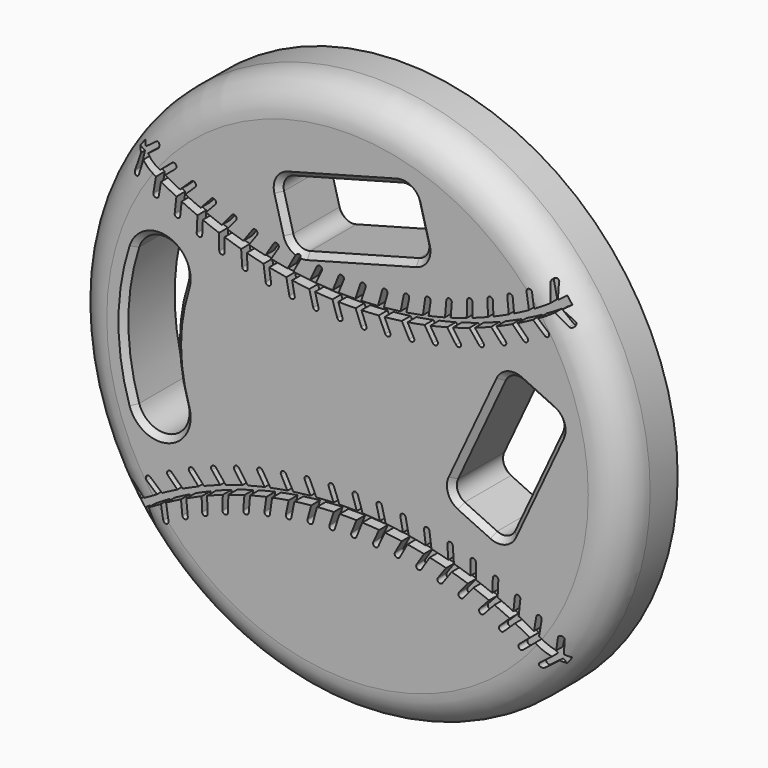
from build123d import *

# Parameters (mm, degrees)
F0_R          = 12.7
F1_DEPTH      = 3.175
F2_SIZE       = 0.254
F5_DEPTH      = 0.508
F7_DEPTH      = 0.508
F9_DEPTH      = 0.508
F14_DEPTH     = 25.4
F15_SIZE      = 0.254
F17_DEPTH     = 25.4
F18_T1_DEPTH  = 1.651
F18_T3_DEPTH  = 5.207
F18_T5_DEPTH  = 1.651
F18_T7_DEPTH  = 5.207
F18_T10_ANGLE = 90
F18_T12_ANGLE = 90
F18_T14_ANGLE = 90
F18_T16_ANGLE = 90
F18_T18_ANGLE = 90
F18_T20_ANGLE = 90
F18_T22_ANGLE = 90
F18_T24_ANGLE = 90


# Not quite as in the source:
# - a fillet or chamfer that OpenCascade refuses, or shapes differently, is made with other operations: its cross-section is extruded or revolved along the edge and cut away or added
# - ends of sketch curves that miss each other by under 0.0002 mm in the source are joined


with BuildPart() as f1:
    # F0 (on Front) → F1 (new body)
    with BuildSketch(Plane.XZ):
        Circle(F0_R)
        with BuildLine():
            ThreePointArc((-9.818145271, -3.175), (-10.31875, 0), (-9.818145271, 3.175))
            ThreePointArc((-9.818145271, 3.175), (-8.3189362013, 3.941516762), (-7.5524194392, 2.4423076923))
            ThreePointArc((-7.5524194392, 2.4423076923), (-7.9375, 0), (-7.5524194392, -2.4423076923))
            ThreePointArc((-7.5524194392, -2.4423076923), (-8.3189362013, -3.941516762), (-9.818145271, -3.175))
        make_face(mode=Mode.SUBTRACT)
    extrude(amount=F1_DEPTH)

    # F2
    f2_edges = [f1.edges().sort_by_distance(p)[0] for p in [
        (-8.318936, -3.175, -3.941517),
        (-7.9375, -3.175, 0),
        (-7.9375, 0, 0),
    ]]
    chamfer(f2_edges, length=F2_SIZE)

    # F4 (on face) → F5 (cut)
    with BuildSketch(Plane.XZ.offset(3.175)):
        with BuildLine():
            ThreePointArc((10.0903170963, 7.7120361057), (0, 4.4873333333), (-10.0903170963, 7.7120361057))
            ThreePointArc((-10.0903170963, 7.7120361057), (-10.204882315, 7.5597868314), (-10.3171505, 7.4058359123))
            ThreePointArc((-10.3171505, 7.4058359123), (0, 4.1063333333), (10.3171505, 7.4058359123))
            ThreePointArc((10.3171505, 7.4058359123), (10.204882315, 7.5597868314), (10.0903170963, 7.7120361057))
        make_face()
        with BuildLine():
            ThreePointArc((-10.3171505, -7.4058359123), (-10.204882315, -7.5597868314), (-10.0903170963, -7.7120361057))
            ThreePointArc((-10.0903170963, -7.7120361057), (0, -4.4873333333), (10.0903170963, -7.7120361057))
            ThreePointArc((10.0903170963, -7.7120361057), (10.204882315, -7.5597868314), (10.3171505, -7.4058359123))
            ThreePointArc((10.3171505, -7.4058359123), (0, -4.1063333333), (-10.3171505, -7.4058359123))
        make_face()
    extrude(amount=-F5_DEPTH, mode=Mode.SUBTRACT)

    # F6 (on face) → F7 (cut)
    with BuildSketch(Plane.XZ.offset(3.175)):
        with BuildLine():
            Line((8.9655202832, -7.7774051542), (9.7084275034, -7.2188150469))
            ThreePointArc((9.7084275034, -7.2188150469), (9.5954418436, -7.1446517893), (9.481889674, -7.0713588641))
            Line((9.481889674, -7.0713588641), (8.8128738495, -7.5743902131))
            ThreePointArc((8.8128738495, -7.5743902131), (8.7876895958, -7.7522209005), (8.9655202832, -7.7774051542))
        make_face()
        with BuildLine():
            Line((-9.1205047211, -7.8770944945), (-9.3207214809, -6.9694341534))
            ThreePointArc((-9.3207214809, -6.9694341534), (-9.4350615627, -7.0414917261), (-9.5488446034, -7.1144257218))
            Line((-9.5488446034, -7.1144257218), (-9.3685418994, -7.931807913))
            ThreePointArc((-9.3685418994, -7.931807913), (-9.217166601, -8.0284697929), (-9.1205047211, -7.8770944945))
        make_face()
        with BuildLine():
            ThreePointArc((-9.5488446034, -7.1144257218), (-9.4350615627, -7.0414917261), (-9.3207214809, -6.9694341534))
            Line((-9.3207214809, -6.9694341534), (-10.0499520862, -6.4086497383))
            ThreePointArc((-10.0499520862, -6.4086497383), (-10.2280453511, -6.4319046086), (-10.2047904808, -6.6099978735))
            Line((-10.2047904808, -6.6099978735), (-9.5488446034, -7.1144257218))
        make_face()
        with BuildLine():
            Line((-8.2616111371, -7.3540137205), (-8.4068864974, -6.4359564699))
            ThreePointArc((-8.4068864974, -6.4359564699), (-8.5253526153, -6.5010081955), (-8.6433154009, -6.5669682539))
            Line((-8.6433154009, -6.5669682539), (-8.5124894884, -7.3937132522))
            ThreePointArc((-8.5124894884, -7.3937132522), (-8.3672005469, -7.4993026621), (-8.2616111371, -7.3540137205))
        make_face()
        with BuildLine():
            ThreePointArc((-8.6433154009, -6.5669682539), (-8.5253526153, -6.5010081955), (-8.4068864974, -6.4359564699))
            Line((-8.4068864974, -6.4359564699), (-9.1010766453, -5.8323369918))
            ThreePointArc((-9.1010766453, -5.8323369918), (-9.280245996, -5.8448407425), (-9.2677422452, -6.0240100932))
            Line((-9.2677422452, -6.0240100932), (-8.6433154009, -6.5669682539))
        make_face()
        with BuildLine():
            Line((-7.3728180575, -6.8835261579), (-7.4626262541, -5.9583945275))
            ThreePointArc((-7.4626262541, -5.9583945275), (-7.5847896689, -6.0162049781), (-7.7065052817, -6.0749523839))
            Line((-7.7065052817, -6.0749523839), (-7.6256296312, -6.9080681266))
            ThreePointArc((-7.6256296312, -6.9080681266), (-7.48695286, -7.0222029291), (-7.3728180575, -6.8835261579))
        make_face()
        with BuildLine():
            ThreePointArc((-7.7065052817, -6.0749523839), (-7.5847896689, -6.0162049781), (-7.4626262541, -5.9583945275))
            Line((-7.4626262541, -5.9583945275), (-8.1192636096, -5.3141245382))
            ThreePointArc((-8.1192636096, -5.3141245382), (-8.2988606164, -5.3158319172), (-8.2971532374, -5.495428924))
            Line((-8.2971532374, -5.495428924), (-7.7065052817, -6.0749523839))
        make_face()
        with BuildLine():
            Line((-6.4573421027, -6.4673345424), (-6.4913581118, -5.5384766648))
            ThreePointArc((-6.4913581118, -5.5384766648), (-6.6167767033, -5.5888366191), (-6.7418046438, -5.6401587604))
            Line((-6.7418046438, -5.6401587604), (-6.7111719514, -6.4766301285))
            ThreePointArc((-6.7111719514, -6.4766301285), (-6.5796092339, -6.5988972598), (-6.4573421027, -6.4673345424))
        make_face()
        with BuildLine():
            ThreePointArc((-6.7418046438, -5.6401587604), (-6.6167767033, -5.5888366191), (-6.4913581118, -5.5384766648))
            Line((-6.4913581118, -5.5384766648), (-7.1080662467, -4.8558878338))
            ThreePointArc((-7.1080662467, -4.8558878338), (-7.2874409323, -4.8467926619), (-7.2965361041, -5.0261673476))
            Line((-7.2965361041, -5.0261673476), (-6.7418046438, -5.6401587604))
        make_face()
        with BuildLine():
            Line((-5.5184964603, -6.1069451079), (-5.4965971749, -5.1777226012))
            ThreePointArc((-5.4965971749, -5.1777226012), (-5.6248170423, -5.2204498023), (-5.7527048234, -5.2641609397))
            Line((-5.7527048234, -5.2641609397), (-5.7724259515, -6.10096067))
            ThreePointArc((-5.7724259515, -6.10096067), (-5.6484534248, -6.2309176346), (-5.5184964603, -6.1069451079))
        make_face()
        with BuildLine():
            ThreePointArc((-5.7527048234, -5.2641609397), (-5.6248170423, -5.2204498023), (-5.4965971749, -5.1777226012))
            Line((-5.4965971749, -5.1777226012), (-6.0711441684, -4.4592852774))
            ThreePointArc((-6.0711441684, -4.4592852774), (-6.2496473602, -4.439420471), (-6.2695121666, -4.6179236627))
            Line((-6.2695121666, -4.6179236627), (-5.7527048234, -5.2641609397))
        make_face()
        with BuildLine():
            Line((-4.559678895, -5.8036621355), (-4.4819435707, -4.8774379374))
            ThreePointArc((-4.4819435707, -4.8774379374), (-4.612500675, -4.9123777518), (-4.7427854596, -4.9483196908))
            Line((-4.7427854596, -4.9483196908), (-4.8127890357, -5.7824193317))
            ThreePointArc((-4.8127890357, -5.7824193317), (-4.6968553672, -5.9195958039), (-4.559678895, -5.8036621355))
        make_face()
        with BuildLine():
            ThreePointArc((-4.7427854596, -4.9483196908), (-4.612500675, -4.9123777518), (-4.4819435707, -4.8774379374))
            Line((-4.4819435707, -4.8774379374), (-5.0122500868, -4.1257522086))
            ThreePointArc((-5.0122500868, -4.1257522086), (-5.1892357659, -4.09518966), (-5.2197983146, -4.2721753391))
            Line((-5.2197983146, -4.2721753391), (-4.7427854596, -4.9483196908))
        make_face()
        with BuildLine():
            Line((-3.5843594519, -5.5585832327), (-3.4510694196, -4.63870943))
            ThreePointArc((-3.4510694196, -4.63870943), (-3.5834912631, -4.6657354074), (-3.7157015392, -4.6937780711))
            Line((-3.7157015392, -4.6937780711), (-3.8357342141, -5.5221589427))
            ThreePointArc((-3.8357342141, -5.5221589427), (-3.728258978, -5.6660584689), (-3.5843594519, -5.5585832327))
        make_face()
        with BuildLine():
            ThreePointArc((-3.7157015392, -4.6937780711), (-3.5834912631, -4.6657354074), (-3.4510694196, -4.63870943))
            Line((-3.4510694196, -4.63870943), (-3.9352162324, -3.8564957127))
            ThreePointArc((-3.9352162324, -3.8564957127), (-4.1100438722, -3.8153460305), (-4.1511935545, -3.9901736703))
            Line((-4.1511935545, -3.9901736703), (-3.7157015392, -4.6937780711))
        make_face()
        with BuildLine():
            Line((-2.5960678974, -5.3725953618), (-2.4077055454, -4.4624010583))
            ThreePointArc((-2.4077055454, -4.4624010583), (-2.541512882, -4.4814153893), (-2.6751701689, -4.5014572888))
            Line((-2.6751701689, -4.5014572888), (-2.8447975339, -5.3211214082))
            ThreePointArc((-2.8447975339, -5.3211214082), (-2.7461696925, -5.4712232033), (-2.5960678974, -5.3725953618))
        make_face()
        with BuildLine():
            ThreePointArc((-2.6751701689, -4.5014572888), (-2.541512882, -4.4814153893), (-2.4077055454, -4.4624010583))
            Line((-2.4077055454, -4.4624010583), (-2.8439404852, -3.6524902526))
            ThreePointArc((-2.8439404852, -3.6524902526), (-3.0159773692, -3.6009023611), (-3.0675652608, -3.772939245))
            Line((-3.0675652608, -3.772939245), (-2.6751701689, -4.5014572888))
        make_face()
        with BuildLine():
            Line((-1.5983809455, -5.246371629), (-1.3556279737, -4.3491508979))
            ThreePointArc((-1.3556279737, -4.3491508979), (-1.4903365427, -4.360084768), (-1.6249571231, -4.3720533698))
            Line((-1.6249571231, -4.3720533698), (-1.8435652819, -5.1800343006))
            ThreePointArc((-1.8435652819, -5.1800343006), (-1.7541417779, -5.335795133), (-1.5983809455, -5.246371629))
        make_face()
        with BuildLine():
            ThreePointArc((-1.6249571231, -4.3720533698), (-1.4903365427, -4.360084768), (-1.3556279737, -4.3491508979))
            Line((-1.3556279737, -4.3491508979), (-1.742372268, -3.514474142))
            ThreePointArc((-1.742372268, -3.514474142), (-1.9109957795, -3.4526347423), (-1.9728351792, -3.6212582538))
            Line((-1.9728351792, -3.6212582538), (-1.6249571231, -4.3720533698))
        make_face()
        with BuildLine():
            Line((-0.5949093127, -5.1803688492), (-0.2986442654, -4.2993688109))
            ThreePointArc((-0.2986442654, -4.2993688109), (-0.4337665448, -4.3021826495), (-0.5688632149, -4.3060346383))
            Line((-0.5688632149, -4.3060346383), (-0.8356610054, -5.0994082266))
            ThreePointArc((-0.8356610054, -5.0994082266), (-0.7557654704, -5.2602643843), (-0.5949093127, -5.1803688492))
        make_face()
        with BuildLine():
            ThreePointArc((-0.5688632149, -4.3060346383), (-0.4337665448, -4.3021826495), (-0.2986442654, -4.2993688109))
            Line((-0.2986442654, -4.2993688109), (-0.6344982526, -3.4429468734))
            ThreePointArc((-0.6344982526, -3.4429468734), (-0.7990981284, -3.3710797676), (-0.8709652341, -3.5356796434))
            Line((-0.8709652341, -3.5356796434), (-0.5688632149, -4.3060346383))
        make_face()
        with BuildLine():
            Line((0.4107153491, -5.1748258922), (0.7594202627, -4.3132349632))
            ThreePointArc((0.7594202627, -4.3132349632), (0.6243732923, -4.3079185867), (0.4892894591, -4.3036400218))
            Line((0.4892894591, -4.3036400218), (0.1752676015, -5.0795349789))
            ThreePointArc((0.1752676015, -5.0795349789), (0.2453460187, -5.2449043094), (0.4107153491, -5.1748258922))
        make_face()
        with BuildLine():
            ThreePointArc((0.4892894591, -4.3036400218), (0.6243732923, -4.3079185867), (0.7594202627, -4.3132349632))
            Line((0.7594202627, -4.3132349632), (0.4756720676, -3.43816731))
            ThreePointArc((0.4756720676, -3.43816731), (0.3156915289, -3.3565325916), (0.2340568106, -3.5165131303))
            Line((0.2340568106, -3.5165131303), (0.4892894591, -4.3036400218))
        make_face()
        with BuildLine():
            Line((1.414853596, -5.2297628184), (1.8147363823, -4.3906991719))
            ThreePointArc((1.8147363823, -4.3906991719), (1.6802534676, -4.3772718207), (1.5456713517, -4.3648781866))
            Line((1.5456713517, -4.3648781866), (1.1855618997, -5.1204864807))
            ThreePointArc((1.1855618997, -5.1204864807), (1.245569579, -5.2897704977), (1.414853596, -5.2297628184))
        make_face()
        with BuildLine():
            ThreePointArc((1.5456713517, -4.3648781866), (1.6802534676, -4.3772718207), (1.8147363823, -4.3906991719))
            Line((1.8147363823, -4.3906991719), (1.5841208889, -3.5001527497))
            ThreePointArc((1.5841208889, -3.5001527497), (1.4293386709, -3.4090458619), (1.3382317831, -3.5638280798))
            Line((1.3382317831, -3.5638280798), (1.5456713517, -4.3648781866))
        make_face()
        with BuildLine():
            Line((2.4138713637, -5.3449808064), (2.8634848117, -4.5314810872))
            ThreePointArc((2.8634848117, -4.5314810872), (2.7300526583, -4.5099913561), (2.5964593241, -4.4895275065))
            Line((2.5964593241, -4.4895275065), (2.1915655453, -5.2221145249))
            ThreePointArc((2.1915655453, -5.2221145249), (2.2412853137, -5.3947005748), (2.4138713637, -5.3449808064))
        make_face()
        with BuildLine():
            ThreePointArc((2.5964593241, -4.4895275065), (2.7300526583, -4.5099913561), (2.8634848117, -4.5314810872))
            Line((2.8634848117, -4.5314810872), (2.6868366377, -3.6286788616))
            ThreePointArc((2.6868366377, -3.6286788616), (2.5378129109, -3.5284295282), (2.4375635775, -3.677453255))
            Line((2.4375635775, -3.677453255), (2.5964593241, -4.4895275065))
        make_face()
        with BuildLine():
            Line((3.4041531191, -5.520062872), (3.9018700383, -4.7350712071))
            ThreePointArc((3.9018700383, -4.7350712071), (3.7699715489, -4.7055968693), (3.6378504824, -4.6771368646))
            Line((3.6378504824, -4.6771368646), (3.189637723, -5.3840513105))
            ThreePointArc((3.189637723, -5.3840513105), (3.2288896403, -5.5593147893), (3.4041531191, -5.520062872))
        make_face()
        with BuildLine():
            ThreePointArc((3.6378504824, -4.6771368646), (3.7699715489, -4.7055968693), (3.9018700383, -4.7350712071))
            Line((3.9018700383, -4.7350712071), (3.779828489, -3.8232804985))
            ThreePointArc((3.779828489, -3.8232804985), (3.6371025833, -3.7142515307), (3.5280736154, -3.8569774364))
            Line((3.5280736154, -3.8569774364), (3.6378504824, -4.6771368646))
        make_face()
        with BuildLine():
            Line((4.3821149457, -5.7543753779), (4.926134055, -5.0007327209))
            ThreePointArc((4.926134055, -5.0007327209), (4.7962465817, -4.9633804468), (4.6660759406, -4.9270272862))
            Line((4.6660759406, -4.9270272862), (4.1761663219, -5.6057107743))
            ThreePointArc((4.1761663219, -5.6057107743), (4.204808332, -5.783017388), (4.3821149457, -5.7543753779))
        make_face()
        with BuildLine():
            ThreePointArc((4.6660759406, -4.9270272862), (4.7962465817, -4.9633804468), (4.926134055, -5.0007327209))
            Line((4.926134055, -5.0007327209), (4.8591408094, -4.0832533801))
            ThreePointArc((4.8591408094, -4.0832533801), (4.7232292623, -3.9658393631), (4.6058152454, -4.1017509102))
            Line((4.6058152454, -4.1017509102), (4.6660759406, -4.9270272862))
        make_face()
        with BuildLine():
            Line((5.3442175139, -6.0470703267), (5.9325699604, -5.3275041765))
            ThreePointArc((5.9325699604, -5.3275041765), (5.8051635774, -5.2824091471), (5.6774144607, -5.2382943959))
            Line((5.6774144607, -5.2382943959), (5.1475810086, -5.8862907112))
            ThreePointArc((5.1475810086, -5.8862907112), (5.1655094535, -6.0649987716), (5.3442175139, -6.0470703267))
        make_face()
        with BuildLine():
            ThreePointArc((5.6774144607, -5.2382943959), (5.8051635774, -5.2824091471), (5.9325699604, -5.3275041765))
            Line((5.9325699604, -5.3275041765), (5.9208674729, -4.4076566415))
            ThreePointArc((5.9208674729, -4.4076566415), (5.7922621603, -4.2822825071), (5.6668880259, -4.4108878197))
            Line((5.6668880259, -4.4108878197), (5.6774144607, -5.2382943959))
        make_face()
        with BuildLine():
            Line((6.2869788901, -6.3970884296), (6.9175353746, -5.7142029593))
            ThreePointArc((6.9175353746, -5.7142029593), (6.7930711768, -5.6615283774), (6.6682059198, -5.6098116908))
            Line((6.6682059198, -5.6098116908), (6.100366148, -6.2247756777))
            ThreePointArc((6.100366148, -6.2247756777), (6.1075161431, -6.4042384247), (6.2869788901, -6.3970884296))
        make_face()
        with BuildLine():
            ThreePointArc((6.6682059198, -5.6098116908), (6.7930711768, -5.6615283774), (6.9175353746, -5.7142029593))
            Line((6.9175353746, -5.7142029593), (6.9611659976, -4.7953162391))
            ThreePointArc((6.9611659976, -4.7953162391), (6.8403323534, -4.6624357272), (6.7074518416, -4.7832693714))
            Line((6.7074518416, -4.7832693714), (6.6682059198, -5.6098116908))
        make_face()
        with BuildLine():
            Line((7.2069871381, -6.8031629404), (7.8774656214, -6.1594295724))
            ThreePointArc((7.8774656214, -6.1594295724), (7.7563940557, -6.099366072), (7.6348645567, -6.0402346172))
            Line((7.6348645567, -6.0402346172), (7.0310735271, -6.619940667))
            ThreePointArc((7.0310735271, -6.619940667), (7.0274191959, -6.7995086092), (7.2069871381, -6.8031629404))
        make_face()
        with BuildLine():
            ThreePointArc((7.6348645567, -6.0402346172), (7.7563940557, -6.099366072), (7.8774656214, -6.1594295724))
            Line((7.8774656214, -6.1594295724), (7.9762714519, -5.2448291986))
            ThreePointArc((7.9762714519, -5.2448291986), (7.8636467837, -5.1049232155), (7.7237408006, -5.2175478837))
            Line((7.7237408006, -5.2175478837), (7.6348645567, -6.0402346172))
        make_face()
        with BuildLine():
            Line((8.1009126675, -7.2638242398), (8.8088866291, -6.6615727016))
            ThreePointArc((8.8088866291, -6.6615727016), (8.6916458641, -6.5943376578), (8.5738919489, -6.5280054368))
            Line((8.5738919489, -6.5280054368), (7.9363348343, -7.0703555425))
            ThreePointArc((7.9363348343, -7.0703555425), (7.9218894022, -7.2493788077), (8.1009126675, -7.2638242398))
        make_face()
        with BuildLine():
            ThreePointArc((8.5738919489, -6.5280054368), (8.6916458641, -6.5943376578), (8.8088866291, -6.6615727016))
            Line((8.8088866291, -6.6615727016), (8.9625100801, -5.7545686932))
            ThreePointArc((8.9625100801, -5.7545686932), (8.8585019863, -5.6081435709), (8.7120768641, -5.7121516647))
            Line((8.7120768641, -5.7121516647), (8.5738919489, -6.5280054368))
        make_face()
        with BuildLine():
            ThreePointArc((9.481889674, -7.0713588641), (9.5954418436, -7.1446517893), (9.7084275034, -7.2188150469))
            Line((9.7084275034, -7.2188150469), (9.916312598, -6.322689931))
            ThreePointArc((9.916312598, -6.322689931), (9.8212974932, -6.1702755949), (9.6688831571, -6.2652906998))
            Line((9.6688831571, -6.2652906998), (9.481889674, -7.0713588641))
        make_face()
    extrude(amount=-F7_DEPTH, mode=Mode.SUBTRACT)

    # F8 (on face) → F9 (cut)
    with BuildSketch(Plane.XZ.offset(3.175)):
        with BuildLine():
            Line((-8.9656531004, 7.7774905851), (-9.7085603205, 7.2189004778))
            ThreePointArc((-9.7085603205, 7.2189004778), (-9.5955741895, 7.1447379357), (-9.4820226835, 7.0714439946))
            Line((-9.4820226835, 7.0714439946), (-8.8130066667, 7.574475644))
            ThreePointArc((-8.8130066667, 7.574475644), (-8.787822413, 7.7523063314), (-8.9656531004, 7.7774905851))
        make_face()
        with BuildLine():
            ThreePointArc((-9.4820226835, 7.0714439946), (-9.5955741895, 7.1447379357), (-9.7085591779, 7.218902204))
            Line((-9.7085591779, 7.218902204), (-9.9164454152, 6.3227753619))
            ThreePointArc((-9.9164454152, 6.3227753619), (-9.8214303103, 6.1703610258), (-9.6690159742, 6.2653761307))
            Line((-9.6690159742, 6.2653761307), (-9.4820226835, 7.0714439946))
        make_face()
        with BuildLine():
            Line((9.1205047211, 7.8770944945), (9.3207214809, 6.9694341534))
            ThreePointArc((9.3207214809, 6.9694341534), (9.4350615627, 7.0414917261), (9.5488446034, 7.1144257218))
            Line((9.5488446034, 7.1144257218), (9.3685418994, 7.931807913))
            ThreePointArc((9.3685418994, 7.931807913), (9.217166601, 8.0284697929), (9.1205047211, 7.8770944945))
        make_face()
        with BuildLine():
            ThreePointArc((9.5488446034, 7.1144257218), (9.4350615627, 7.0414917261), (9.3207214809, 6.9694341534))
            Line((9.3207214809, 6.9694341534), (10.0499520862, 6.4086497383))
            ThreePointArc((10.0499520862, 6.4086497383), (10.2280453511, 6.4319046086), (10.2047904808, 6.6099978735))
            Line((10.2047904808, 6.6099978735), (9.5488446034, 7.1144257218))
        make_face()
        with BuildLine():
            Line((8.2616023603, 7.3540139847), (8.4068777206, 6.435956734))
            ThreePointArc((8.4068777206, 6.435956734), (8.5253460125, 6.5010045368), (8.6433088565, 6.5669645615))
            Line((8.6433088565, 6.5669645615), (8.5124807117, 7.3937135163))
            ThreePointArc((8.5124807117, 7.3937135163), (8.3671917702, 7.4993029262), (8.2616023603, 7.3540139847))
        make_face()
        with BuildLine():
            ThreePointArc((8.6433088565, 6.5669645615), (8.5253460125, 6.5010045368), (8.4068798364, 6.4359528455))
            Line((8.4068798364, 6.4359528455), (9.1010678685, 5.8323372559))
            ThreePointArc((9.1010678685, 5.8323372559), (9.2802372192, 5.8448410067), (9.2677334684, 6.0240103573))
            Line((9.2677334684, 6.0240103573), (8.6433088565, 6.5669645615))
        make_face()
        with BuildLine():
            Line((7.3728005358, 6.8835272134), (7.4626087323, 5.9583955831))
            ThreePointArc((7.4626087323, 5.9583955831), (7.5847758163, 6.0161983575), (7.7064915391, 6.0749456857))
            Line((7.7064915391, 6.0749456857), (7.6256121094, 6.9080691821))
            ThreePointArc((7.6256121094, 6.9080691821), (7.4869353383, 7.0222039846), (7.3728005358, 6.8835272134))
        make_face()
        with BuildLine():
            ThreePointArc((7.7064915391, 6.0749456857), (7.5847758163, 6.0161983575), (7.4626122919, 5.9583879858))
            Line((7.4626122919, 5.9583879858), (8.1192460879, 5.3141255937))
            ThreePointArc((8.1192460879, 5.3141255937), (8.2988430947, 5.3158329727), (8.2971357156, 5.4954299795))
            Line((8.2971357156, 5.4954299795), (7.7064915391, 6.0749456857))
        make_face()
        with BuildLine():
            Line((6.4573158993, 6.4673369137), (6.4913319084, 5.5384790361))
            ThreePointArc((6.4913319084, 5.5384790361), (6.6167550351, 5.5888278218), (6.7417831294, 5.6401498324))
            Line((6.7417831294, 5.6401498324), (6.711145748, 6.4766324999))
            ThreePointArc((6.711145748, 6.4766324999), (6.5795830306, 6.5988996311), (6.4573158993, 6.4673369137))
        make_face()
        with BuildLine():
            ThreePointArc((6.7417831294, 5.6401498324), (6.6167550351, 5.5888278218), (6.4913362906, 5.538468))
            Line((6.4913362906, 5.538468), (7.1080400433, 4.8558902051))
            ThreePointArc((7.1080400433, 4.8558902051), (7.287414729, 4.8467950333), (7.2965099008, 5.0261697189))
            Line((7.2965099008, 5.0261697189), (6.7417831294, 5.6401498324))
        make_face()
        with BuildLine():
            Line((5.5184616702, 6.1069493147), (5.4965623848, 5.177726808))
            ThreePointArc((5.4965623848, 5.177726808), (5.6247870854, 5.2204396916), (5.7526750548, 5.2641506371))
            Line((5.7526750548, 5.2641506371), (5.7723911614, 6.1009648768))
            ThreePointArc((5.7723911614, 6.1009648768), (5.6484186347, 6.2309218414), (5.5184616702, 6.1069493147))
        make_face()
        with BuildLine():
            ThreePointArc((5.7526750548, 5.2641506371), (5.6247870854, 5.2204396916), (5.496567031, 5.1777126847))
            Line((5.496567031, 5.1777126847), (6.0711093783, 4.4592894842))
            ThreePointArc((6.0711093783, 4.4592894842), (6.2496125701, 4.4394246778), (6.2694773765, 4.6179278695))
            Line((6.2694773765, 4.6179278695), (5.7526750548, 5.2641506371))
        make_face()
        with BuildLine():
            Line((4.5596356441, 5.8036686908), (4.4819003198, 4.8774444927))
            ThreePointArc((4.4819003198, 4.8774444927), (4.6124620582, 4.912367258), (4.7427470553, 4.9483089373))
            Line((4.7427470553, 4.9483089373), (4.8127457847, 5.782425887))
            ThreePointArc((4.8127457847, 5.782425887), (4.6968121163, 5.9196023592), (4.5596356441, 5.8036686908))
        make_face()
        with BuildLine():
            ThreePointArc((4.7427470553, 4.9483089373), (4.6124620582, 4.912367258), (4.4819047432, 4.8774277061))
            Line((4.4819047432, 4.8774277061), (5.0122068359, 4.1257587639))
            ThreePointArc((5.0122068359, 4.1257587639), (5.189192515, 4.0951962153), (5.2197550636, 4.2721818944))
            Line((5.2197550636, 4.2721818944), (4.7427470553, 4.9483089373))
        make_face()
        with BuildLine():
            Line((3.5843078966, 5.5585926411), (3.4510178643, 4.6387188383))
            ThreePointArc((3.4510178643, 4.6387188383), (3.5834437256, 4.6657255151), (3.7156542272, 4.6937678458))
            Line((3.7156542272, 4.6937678458), (3.8356826588, 5.522168351))
            ThreePointArc((3.8356826588, 5.522168351), (3.7282074227, 5.6660678772), (3.5843078966, 5.5585926411))
        make_face()
        with BuildLine():
            ThreePointArc((3.7156542272, 4.6937678458), (3.5834437256, 4.6657255151), (3.4510216589, 4.6386998736))
            Line((3.4510216589, 4.6386998736), (3.9351646771, 3.856505121))
            ThreePointArc((3.9351646771, 3.856505121), (4.109992317, 3.8153554388), (4.1511419992, 3.9901830786))
            Line((4.1511419992, 3.9901830786), (3.7156542272, 4.6937678458))
        make_face()
        with BuildLine():
            Line((2.5960082244, 5.3726081173), (2.4076458724, 4.4624138138))
            ThreePointArc((2.4076458724, 4.4624138138), (2.5414562801, 4.4814071242), (2.6751137936, 4.5014486138))
            Line((2.6751137936, 4.5014486138), (2.8447378609, 5.3211341637))
            ThreePointArc((2.8447378609, 5.3211341637), (2.7461100195, 5.4712359588), (2.5960082244, 5.3726081173))
        make_face()
        with BuildLine():
            ThreePointArc((2.6751137936, 4.5014486138), (2.5414562801, 4.4814071242), (2.40764872, 4.462393206))
            Line((2.40764872, 4.462393206), (2.8438808122, 3.6525030081))
            ThreePointArc((2.8438808122, 3.6525030081), (3.0159176962, 3.6009151166), (3.0675055878, 3.7729520006))
            Line((3.0675055878, 3.7729520006), (2.6751137936, 4.5014486138))
        make_face()
        with BuildLine():
            Line((1.5983133707, 5.2463882138), (1.3555603989, 4.3491674827))
            ThreePointArc((1.3555603989, 4.3491674827), (1.4902708551, 4.3600791823), (1.6248916506, 4.3720472954))
            Line((1.6248916506, 4.3720472954), (1.8434977072, 5.1800508854))
            ThreePointArc((1.8434977072, 5.1800508854), (1.7540742031, 5.3358117178), (1.5983133707, 5.2463882138))
        make_face()
        with BuildLine():
            ThreePointArc((1.6248916506, 4.3720472954), (1.4902708551, 4.3600791823), (1.3555620746, 4.3491458039))
            Line((1.3555620746, 4.3491458039), (1.7423046932, 3.5144907268))
            ThreePointArc((1.7423046932, 3.5144907268), (1.9109282047, 3.4526513271), (1.9727676045, 3.6212748386))
            Line((1.9727676045, 3.6212748386), (1.6248916506, 4.3720472954))
        make_face()
        with BuildLine():
            Line((0.5948340807, 5.1803897315), (0.2985690334, 4.2993896932))
            ThreePointArc((0.2985690334, 4.2993896932), (0.4336918755, 4.3021808077), (0.5687887366, 4.3060322285))
            Line((0.5687887366, 4.3060322285), (0.8355857735, 5.0994291088))
            ThreePointArc((0.8355857735, 5.0994291088), (0.7556902384, 5.2602852666), (0.5948340807, 5.1803897315))
        make_face()
        with BuildLine():
            ThreePointArc((0.5687887366, 4.3060322285), (0.4336918755, 4.3021808077), (0.2985694095, 4.2993675399))
            Line((0.2985694095, 4.2993675399), (0.6344230206, 3.4429677556))
            ThreePointArc((0.6344230206, 3.4429677556), (0.7990228964, 3.3711006499), (0.8708900022, 3.5357005257))
            Line((0.8708900022, 3.5357005257), (0.5687887366, 4.3060322285))
        make_face()
        with BuildLine():
            Line((-0.4107979661, 5.1748515246), (-0.7595028797, 4.3132605956))
            ThreePointArc((-0.7595028797, 4.3132605956), (-0.624456712, 4.3079215499), (-0.489372725, 4.3036423391))
            Line((-0.489372725, 4.3036423391), (-0.1753502185, 5.0795606114))
            ThreePointArc((-0.1753502185, 5.0795606114), (-0.2454286356, 5.2449299418), (-0.4107979661, 5.1748515246))
        make_face()
        with BuildLine():
            ThreePointArc((-0.489372725, 4.3036423391), (-0.624456712, 4.3079215499), (-0.7595038314, 4.3132385748))
            Line((-0.7595038314, 4.3132385748), (-0.4757546845, 3.4381929424))
            ThreePointArc((-0.4757546845, 3.4381929424), (-0.3157741459, 3.3565582241), (-0.2341394275, 3.5165387627))
            Line((-0.2341394275, 3.5165387627), (-0.489372725, 4.3036423391))
        make_face()
        with BuildLine():
            Line((-1.4149432989, 5.2297936365), (-1.8148260852, 4.3907299899))
            ThreePointArc((-1.8148260852, 4.3907299899), (-1.6803452798, 4.3772806318), (-1.5457630596, 4.364886277))
            Line((-1.5457630596, 4.364886277), (-1.1856516026, 5.1205172988))
            ThreePointArc((-1.1856516026, 5.1205172988), (-1.2456592819, 5.2898013158), (-1.4149432989, 5.2297936365))
        make_face()
        with BuildLine():
            ThreePointArc((-1.5457630596, 4.364886277), (-1.6803452798, 4.3772806318), (-1.814828293, 4.3907087056))
            Line((-1.814828293, 4.3907087056), (-1.5842105917, 3.5001835677))
            ThreePointArc((-1.5842105917, 3.5001835677), (-1.4294283738, 3.4090766799), (-1.338321486, 3.5638588979))
            Line((-1.338321486, 3.5638588979), (-1.5457630596, 4.364886277))
        make_face()
        with BuildLine():
            Line((-2.4139678278, 5.3450172268), (-2.8635812758, 4.5315175076))
            ThreePointArc((-2.8635812758, 4.5315175076), (-2.7301523801, 4.5100070242), (-2.5965590036, 4.489542384))
            Line((-2.5965590036, 4.489542384), (-2.1916620095, 5.2221509453))
            ThreePointArc((-2.1916620095, 5.2221509453), (-2.2413817779, 5.3947369952), (-2.4139678278, 5.3450172268))
        make_face()
        with BuildLine():
            ThreePointArc((-2.5965590036, 4.489542384), (-2.7301523801, 4.5100070242), (-2.8635845694, 4.5314975473))
            Line((-2.8635845694, 4.5314975473), (-2.6869331018, 3.628715282))
            ThreePointArc((-2.6869331018, 3.628715282), (-2.537909375, 3.5284659486), (-2.4376600416, 3.6774896754))
            Line((-2.4376600416, 3.6774896754), (-2.5965590036, 4.489542384))
        make_face()
        with BuildLine():
            Line((-3.4042559954, 5.5201052911), (-3.9019729147, 4.7351136262))
            ThreePointArc((-3.9019729147, 4.7351136262), (-3.7700785767, 4.705620355), (-3.6379575417, 4.6771594964))
            Line((-3.6379575417, 4.6771594964), (-3.1897405993, 5.3840937297))
            ThreePointArc((-3.1897405993, 5.3840937297), (-3.2289925167, 5.5593572085), (-3.4042559954, 5.5201052911))
        make_face()
        with BuildLine():
            ThreePointArc((-3.6379575417, 4.6771594964), (-3.7700785767, 4.705620355), (-3.9019770277, 4.7350955474))
            Line((-3.9019770277, 4.7350955474), (-3.7799313653, 3.8233229177))
            ThreePointArc((-3.7799313653, 3.8233229177), (-3.6372054596, 3.7142939498), (-3.5281764917, 3.8570198555))
            Line((-3.5281764917, 3.8570198555), (-3.6379575417, 4.6771594964))
        make_face()
        with BuildLine():
            Line((-4.3822238619, 5.7544241706), (-4.9262429712, 5.0007815136))
            ThreePointArc((-4.9262429712, 5.0007815136), (-4.7963601968, 4.9634126479), (-4.666189672, 4.9270585782))
            Line((-4.666189672, 4.9270585782), (-4.1762752381, 5.605759567))
            ThreePointArc((-4.1762752381, 5.605759567), (-4.2049172482, 5.7830661806), (-4.3822238619, 5.7544241706))
        make_face()
        with BuildLine():
            ThreePointArc((-4.666189672, 4.9270585782), (-4.7963601968, 4.9634126479), (-4.9262475465, 5.0007658312))
            Line((-4.9262475465, 5.0007658312), (-4.8592497256, 4.0833021727))
            ThreePointArc((-4.8592497256, 4.0833021727), (-4.7233381785, 3.9658881558), (-4.6059241616, 4.1017997028))
            Line((-4.6059241616, 4.1017997028), (-4.666189672, 4.9270585782))
        make_face()
        with BuildLine():
            Line((-5.3443320758, 6.0471258445), (-5.9326845223, 5.3275596943))
            ThreePointArc((-5.9326845223, 5.3275596943), (-5.8052829534, 5.2824508849), (-5.6775340477, 5.238335179))
            Line((-5.6775340477, 5.238335179), (-5.1476955705, 5.8863462289))
            ThreePointArc((-5.1476955705, 5.8863462289), (-5.1656240154, 6.0650542894), (-5.3443320758, 6.0471258445))
        make_face()
        with BuildLine():
            ThreePointArc((-5.6775340477, 5.238335179), (-5.8052829534, 5.2824508849), (-5.9326891177, 5.3275468682))
            Line((-5.9326891177, 5.3275468682), (-5.9209820348, 4.4077121593))
            ThreePointArc((-5.9209820348, 4.4077121593), (-5.7923767222, 4.2823380249), (-5.6670025878, 4.4109433375))
            Line((-5.6670025878, 4.4109433375), (-5.6775340477, 5.238335179))
        make_face()
        with BuildLine():
            Line((-6.2870986831, 6.3971509998), (-6.9176551676, 5.7142655295))
            ThreePointArc((-6.9176551676, 5.7142655295), (-6.7931953885, 5.6615803839), (-6.668330446, 5.6098627081))
            Line((-6.668330446, 5.6098627081), (-6.100485941, 6.2248382479))
            ThreePointArc((-6.100485941, 6.2248382479), (-6.1076359361, 6.4043009949), (-6.2870986831, 6.3971509998))
        make_face()
        with BuildLine():
            ThreePointArc((-6.668330446, 5.6098627081), (-6.7931953885, 5.6615803839), (-6.9176592639, 5.7142559533))
            Line((-6.9176592639, 5.7142559533), (-6.9612857906, 4.7953788093))
            ThreePointArc((-6.9612857906, 4.7953788093), (-6.8404521464, 4.6624982974), (-6.7075716346, 4.7833319416))
            Line((-6.7075716346, 4.7833319416), (-6.668330446, 5.6098627081))
        make_face()
        with BuildLine():
            Line((-7.2071117287, 6.8032328649), (-7.877590212, 6.1594994968))
            ThreePointArc((-7.877590212, 6.1594994968), (-7.7565220898, 6.0994289785), (-7.6349930162, 6.040296512))
            Line((-7.6349930162, 6.040296512), (-7.0311981176, 6.6200105915))
            ThreePointArc((-7.0311981176, 6.6200105915), (-7.0275437865, 6.7995785337), (-7.2071117287, 6.8032328649))
        make_face()
        with BuildLine():
            ThreePointArc((-7.6349930162, 6.040296512), (-7.7565220898, 6.0994289785), (-7.8775932221, 6.1594934876))
            Line((-7.8775932221, 6.1594934876), (-7.9763960425, 5.244899123))
            ThreePointArc((-7.9763960425, 5.244899123), (-7.8637713742, 5.10499314), (-7.7238653911, 5.2176178082))
            Line((-7.7238653911, 5.2176178082), (-7.6349930162, 6.040296512))
        make_face()
        with BuildLine():
            Line((-8.1010416046, 7.2639017937), (-8.8090155663, 6.6616502555))
            ThreePointArc((-8.8090155663, 6.6616502555), (-8.6917766307, 6.5944119842), (-8.5740232578, 6.5280787423))
            Line((-8.5740232578, 6.5280787423), (-7.9364637715, 7.0704330964))
            ThreePointArc((-7.9364637715, 7.0704330964), (-7.9220183394, 7.2494563616), (-8.1010416046, 7.2639017937))
        make_face()
        with BuildLine():
            ThreePointArc((-8.5740232578, 6.5280787423), (-8.6917766307, 6.5944119842), (-8.8090168454, 6.6616480448))
            Line((-8.8090168454, 6.6616480448), (-8.9626390173, 5.7546462471))
            ThreePointArc((-8.9626390173, 5.7546462471), (-8.8586309235, 5.6082211248), (-8.7122058012, 5.7122292186))
            Line((-8.7122058012, 5.7122292186), (-8.5740232578, 6.5280787423))
        make_face()
    extrude(amount=-F9_DEPTH, mode=Mode.SUBTRACT)

    # F10 (on Top) → F12 (revolve, cut)
    with BuildSketch(Plane.XY):
        with BuildLine():
            ThreePointArc((-11.1125, -3.175), (-12.2350320151, -2.7100320151), (-12.7, -1.5875))
            Line((-12.7, -1.5875), (-12.7, -3.175))
            Line((-12.7, -3.175), (-11.1125, -3.175))
        make_face()
    revolve(axis=Axis((0, -1.5875, 0), (0, -1, 0)), mode=Mode.SUBTRACT)

    # F13 (on face) → F14 (cut)
    with BuildSketch(Plane.XZ.offset(3.175)):
        with BuildLine():
            ThreePointArc((7.94584785, 3.5697929404), (7.4603024628, 3.5909923099), (7.101979809, 3.2626500919))
            Line((7.101979809, 3.2626500919), (4.9014065202, -1.4564945552))
            ThreePointArc((4.9014065202, -1.4564945552), (4.8802071507, -1.9420399424), (5.2085493687, -2.3003625962))
            Line((5.2085493687, -2.3003625962), (6.7048635251, -2.9981053463))
            ThreePointArc((6.7048635251, -2.9981053463), (7.1904089123, -3.0193047158), (7.5487315661, -2.6909624978))
            Line((7.5487315661, -2.6909624978), (9.749304855, 2.0281821493))
            ThreePointArc((9.749304855, 2.0281821493), (9.7705042244, 2.5137275365), (9.4421620064, 2.8720501903))
            Line((9.4421620064, 2.8720501903), (7.94584785, 3.5697929404))
        make_face()
    extrude(amount=-F14_DEPTH, mode=Mode.SUBTRACT)

    # F15
    f15_edges = [f1.edges().sort_by_distance(p)[0] for p in [
        (6.001693, -3.175, 0.903078),
        (6.001693, 0, 0.903078),
    ]]
    chamfer(f15_edges, length=F15_SIZE)

    # F16 (on face) → F17 (cut)
    with BuildSketch(Plane.XZ.offset(3.175)):
        with BuildLine():
            Line((2.3469282464, 9.7537911929), (-2.6826475311, 8.4061204251))
            ThreePointArc((-2.6826475311, 8.4061204251), (-3.0682235688, 8.1102575254), (-3.1316603371, 7.6284074317))
            Line((-3.1316603371, 7.6284074317), (-2.7043500936, 6.0336638925))
            ThreePointArc((-2.7043500936, 6.0336638925), (-2.4084871939, 5.6480878548), (-1.9266371003, 5.5846510865))
            Line((-1.9266371003, 5.5846510865), (3.1029386772, 6.9323218543))
            ThreePointArc((3.1029386772, 6.9323218543), (3.4885147149, 7.228184754), (3.5519514832, 7.7100348477))
            Line((3.5519514832, 7.7100348477), (3.1246412398, 9.3047783869))
            ThreePointArc((3.1246412398, 9.3047783869), (2.8287783401, 9.6903544246), (2.3469282464, 9.7537911929))
        make_face()
    extrude(amount=-F17_DEPTH, mode=Mode.SUBTRACT)

    # F18: chamfer of 0.254 on 2 edges, made by hand

    # F18_s2 → F18_t1 (cut)
    with BuildSketch(Plane(origin=(-2.1168833225, 0, 7.9003161133), x_dir=(0, 1, 0), z_dir=(0.2588190451, 0, -0.9659258263))):
        Polygon((-2.921, -1.0505744716), (-3.175, -1.3045744716), (-3.175, -1.0505744716), align=None)
        Polygon((0, -1.3045744716), (-0.254, -1.0505744716), (0, -1.0505744716), align=None)
    extrude(amount=F18_T1_DEPTH, mode=Mode.SUBTRACT)

    # F18_s4 → F18_t3 (cut)
    with BuildSketch(Plane(origin=(-0.4014141149, 0, -0.1075585879), x_dir=(0, 1, 0), z_dir=(0.9659258263, 0, 0.2588190451))):
        Polygon((0, 5.6390090898), (-0.254, 5.8930090898), (0, 5.8930090898), align=None)
        Polygon((-2.921, 5.8930090898), (-3.175, 5.6390090898), (-3.175, 5.8930090898), align=None)
    extrude(amount=F18_T3_DEPTH, mode=Mode.SUBTRACT)

    # F18_s6 → F18_t5 (cut)
    with BuildSketch(Plane(origin=(-1.689573079, 0, 6.3055725741), x_dir=(0, 1, 0), z_dir=(-0.2588190451, 0, 0.9659258263))):
        Polygon((0, -5.6804255284), (-0.254, -5.4264255284), (0, -5.4264255284), align=None)
        Polygon((-2.921, -5.4264255284), (-3.175, -5.6804255284), (-3.175, -5.4264255284), align=None)
    extrude(amount=F18_T5_DEPTH, mode=Mode.SUBTRACT)

    # F18_s8 → F18_t7 (cut)
    with BuildSketch(Plane(origin=(4.6281616626, 0, 1.2401121799), x_dir=(0, 1, 0), z_dir=(-0.9659258263, 0, -0.2588190451))):
        Polygon((0, -9.0680090898), (-0.254, -8.8140090898), (0, -8.8140090898), align=None)
        Polygon((-2.921, -8.8140090898), (-3.175, -9.0680090898), (-3.175, -8.8140090898), align=None)
    extrude(amount=F18_T7_DEPTH, mode=Mode.SUBTRACT)

    # F18_s9 → F18_t10 (revolve, cut)
    with BuildSketch(Plane(origin=(-1.689573079, 0, 6.3055725741), x_dir=(0, 1, 0), z_dir=(-0.2588190451, 0, 0.9659258263))):
        Polygon((0, 1.3045744716), (-0.254, 1.0505744716), (0, 1.0505744716), align=None)
    revolve(axis=Axis((-2.0909871939, 0, 6.1980139862), (0, -1, 0)), revolution_arc=F18_T10_ANGLE, mode=Mode.SUBTRACT)

    # F18_s11 → F18_t12 (revolve, cut)
    with BuildSketch(Plane(origin=(4.6281616626, 0, 1.2401121799), x_dir=(0, 1, 0), z_dir=(-0.9659258263, 0, -0.2588190451))):
        Polygon((0, -5.6390090898), (-0.254, -5.8930090898), (0, -5.8930090898), align=None)
    revolve(axis=Axis((2.9385885835, 0, 7.545684754), (0, -1, 0)), revolution_arc=F18_T12_ANGLE, mode=Mode.SUBTRACT)

    # F18_s13 → F18_t14 (revolve, cut)
    with BuildSketch(Plane(origin=(-2.1168833225, 0, 7.9003161133), x_dir=(0, 1, 0), z_dir=(0.2588190451, 0, -0.9659258263))):
        Polygon((0, 5.6804255284), (-0.254, 5.4264255284), (0, 5.4264255284), align=None)
    revolve(axis=Axis((2.5112783401, 0, 9.1404282932), (0, -1, 0)), revolution_arc=F18_T14_ANGLE, mode=Mode.SUBTRACT)

    # F18_s15 → F18_t16 (revolve, cut)
    with BuildSketch(Plane(origin=(-0.4014141149, 0, -0.1075585879), x_dir=(0, 1, 0), z_dir=(0.9659258263, 0, 0.2588190451))):
        Polygon((0, 9.0680090898), (-0.254, 8.8140090898), (0, 8.8140090898), align=None)
    revolve(axis=Axis((-2.5182974374, 0, 7.7927575254), (0, -1, 0)), revolution_arc=F18_T16_ANGLE, mode=Mode.SUBTRACT)

    # F18_s17 → F18_t18 (revolve, cut)
    with BuildSketch(Plane(origin=(-0.4014141149, 0, -0.1075585879), x_dir=(0, 1, 0), z_dir=(0.9659258263, 0, 0.2588190451))):
        Polygon((-2.921, 8.8140090898), (-3.175, 9.0680090898), (-3.175, 8.8140090898), align=None)
    revolve(axis=Axis((-2.5182974374, -3.175, 7.7927575254), (0, -1, 0)), revolution_arc=F18_T18_ANGLE, mode=Mode.SUBTRACT)

    # F18_s19 → F18_t20 (revolve, cut)
    with BuildSketch(Plane(origin=(-1.689573079, 0, 6.3055725741), x_dir=(0, 1, 0), z_dir=(-0.2588190451, 0, 0.9659258263))):
        Polygon((-2.921, 1.0505744716), (-3.175, 1.3045744716), (-3.175, 1.0505744716), align=None)
    revolve(axis=Axis((-2.0909871939, -3.175, 6.1980139862), (0, -1, 0)), revolution_arc=F18_T20_ANGLE, mode=Mode.SUBTRACT)

    # F18_s21 → F18_t22 (revolve, cut)
    with BuildSketch(Plane(origin=(4.6281616626, 0, 1.2401121799), x_dir=(0, 1, 0), z_dir=(-0.9659258263, 0, -0.2588190451))):
        Polygon((-2.921, -5.8930090898), (-3.175, -5.6390090898), (-3.175, -5.8930090898), align=None)
    revolve(axis=Axis((2.9385885835, -3.175, 7.545684754), (0, -1, 0)), revolution_arc=F18_T22_ANGLE, mode=Mode.SUBTRACT)

    # F18_s23 → F18_t24 (revolve, cut)
    with BuildSketch(Plane(origin=(-2.1168833225, 0, 7.9003161133), x_dir=(0, 1, 0), z_dir=(0.2588190451, 0, -0.9659258263))):
        Polygon((-2.921, 5.4264255284), (-3.175, 5.6804255284), (-3.175, 5.4264255284), align=None)
    revolve(axis=Axis((2.5112783401, -3.175, 9.1404282932), (0, -1, 0)), revolution_arc=F18_T24_ANGLE, mode=Mode.SUBTRACT)


solid = f1.part
